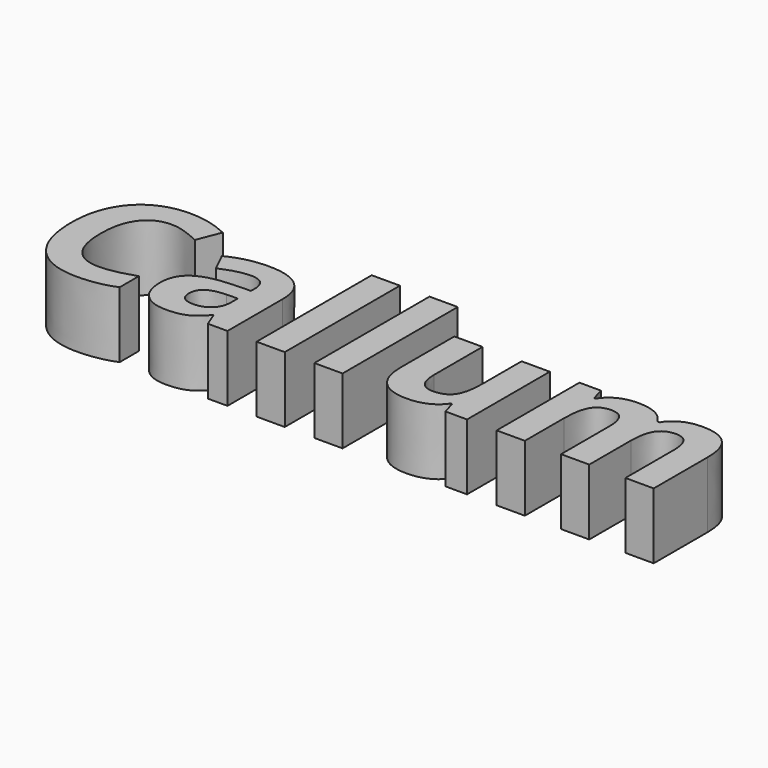
from build123d import *

# Parameters (mm, degrees)
F0_TEXT_SIZE = 71.8025956303
F1_DEPTH     = 25


# Not quite as in the source:
# - Text() gives the source's letters only with a copy of the font that has no kerning and outlines rounded to 1/6400 em; it was checked with that copy


with BuildPart() as f1:
    # F0 (on Top) → F1 (new body)
    with BuildSketch(Plane.XY):
        with Locations((-131.3325315714, -29.5148286968)):
            Text('Callum', F0_TEXT_SIZE, font='Open Sans', font_style=FontStyle.BOLD, text_align=(TextAlign.LEFT, TextAlign.BOTTOM))
    extrude(amount=F1_DEPTH)


solid = f1.part
